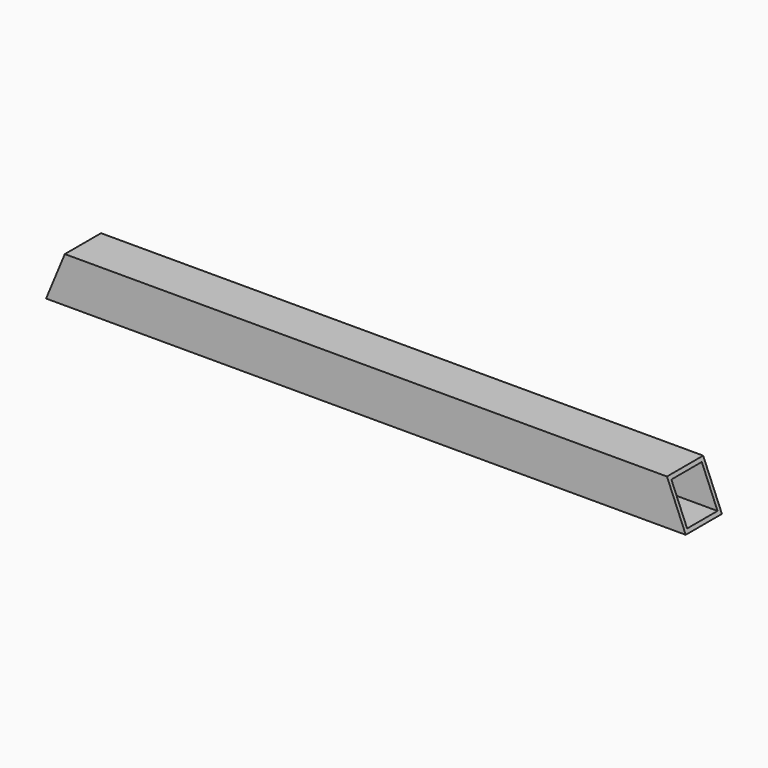
from build123d import *

# Parameters (mm, degrees)
F0_W        = 25
F0_H        = 25
F0_W_2      = 21
F0_H_2      = 21
F1_DEPTH    = 353.347
F2_T1_DEPTH = 154.6335196453
F3_T1_DEPTH = 154.6335196453


# Not quite as in the source:
# - a fillet or chamfer that OpenCascade refuses, or shapes differently, is made with other operations: its cross-section is extruded or revolved along the edge and cut away or added


with BuildPart() as f1:
    # F0 (on Right) → F1 (new body)
    with BuildSketch(Plane.YZ):
        Rectangle(F0_W, F0_H)
        Rectangle(F0_W_2, F0_H_2, mode=Mode.SUBTRACT)
    extrude(amount=F1_DEPTH)

    # F2: chamfer of 25 x 10.3553390593 on 1 edges, made by hand

    # F2_s2 → F2_t1 (cut)
    with BuildSketch(Plane.XZ.offset(-77.3167598227)):
        Polygon((342.9916609407, 12.5), (353.347, -12.5), (353.347, 12.5), align=None)
    extrude(amount=F2_T1_DEPTH, mode=Mode.SUBTRACT)

    # F3: chamfer of 25 x 10.3553390593 on 1 edges, made by hand

    # F3_s2 → F3_t1 (cut)
    with BuildSketch(Plane.XZ.offset(-77.3167598227)):
        Polygon((0, -12.5), (10.3553390593, 12.5), (0, 12.5), align=None)
    extrude(amount=F3_T1_DEPTH, mode=Mode.SUBTRACT)


solid = f1.part
